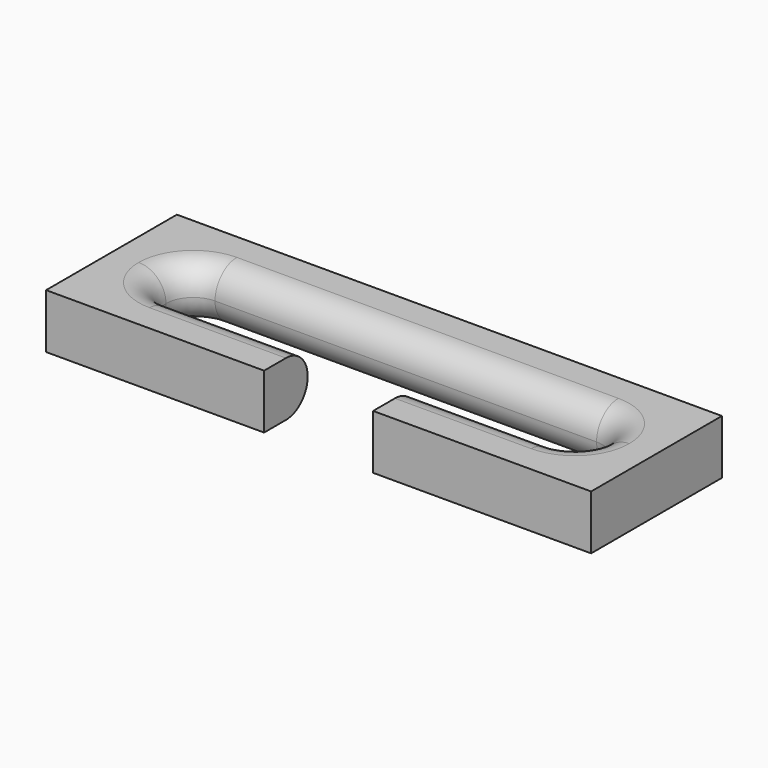
from build123d import *

# Parameters (mm, degrees)
F0_W     = 20
F0_H     = 6
F1_DEPTH = 2
F2_T     = -2
F3_W     = 4
F3_H     = 2
F4_DEPTH = 25
F5_F1_R  = 0.9999
F5_F2_R  = 0.9999


# Not quite as in the source:
# - a fillet or chamfer is up to 0.001 mm smaller than in the source, because OpenCascade refuses the exact size


with BuildPart() as f1:
    # F0 (on Top) → F1 (new body)
    with BuildSketch(Plane.XY):
        with Locations((7.7290598062, 0.812693499)):
            Rectangle(F0_W, F0_H)
    extrude(amount=F1_DEPTH)

    # F2
    f2_openings = [f1.faces().sort_by_distance(p)[0] for p in [
        (7.72906, 0.812693, 2),
        (7.72906, 0.812693, 0),
    ]]
    offset(amount=F2_T, openings=f2_openings)

    # F3 (on face) → F4 (cut)
    with BuildSketch(Plane.XY.offset(2)):
        with Locations((7.7290598062, -1.187306501)):
            Rectangle(F3_W, F3_H)
    extrude(amount=-F4_DEPTH, mode=Mode.SUBTRACT)

    # F5: fillet of radius 1 on 8 edges, made by hand

    # F5_f1 (radius 1 in the source; OpenCascade refuses exactly that, so slightly less here)
    f5_f1_edges = [f1.edges().sort_by_distance(p)[0] for p in [
        (-0.2709401938, 1.812693499, 1),
        (-0.2709401938, -0.187306501, 1),
        (15.7290598062, -0.187306501, 1),
        (15.7290598062, 1.812693499, 1),
    ]]
    fillet(f5_f1_edges, radius=F5_F1_R)

    # F5_f2 (radius 1 in the source; OpenCascade refuses exactly that, so slightly less here)
    f5_f2_edges = [f1.edges().sort_by_distance(p)[0] for p in [
        (-0.2709401938, 0.812693499, 0),
        (-0.2709401938, 0.812693499, 2),
        (15.7290598062, 0.812693499, 0),
        (15.7290598062, 0.812693499, 2),
        (15.4361958767, 0.1055574285, 2),
        (15.4361958767, 1.5198295695, 2),
        (15.4361958767, 0.1055574285, 0),
        (15.4361958767, 1.5198295695, 0),
        (0.0219237357, 1.5198295695, 2),
        (0.0219237357, 0.1055574285, 2),
        (0.0219237357, 1.5198295695, 0),
        (0.0219237357, 0.1055574285, 0),
    ]]
    fillet(f5_f2_edges, radius=F5_F2_R)


solid = f1.part
